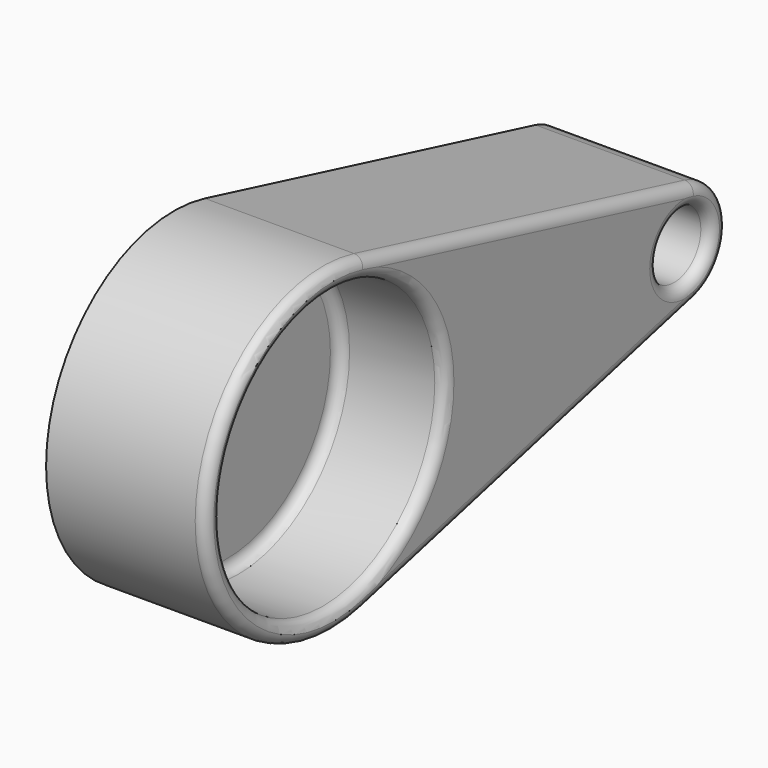
from build123d import *

# Parameters (mm, degrees)
F1_DEPTH    = 76.2
F2_R        = 66.675
F3_DEPTH    = 50.8
F2_R_2      = 15.875
F4_DEPTH    = 50.8
F5_T        = -2.54
F6_T1_DEPTH = 203.2
F6_T3_DEPTH = 203.2
F6_T6_ANGLE = 208.0724869359
F6_T8_ANGLE = 151.9275130641
F7_R        = 5.08
F8_DEPTH    = 25.4


# Not quite as in the source:
# - a fillet or chamfer that OpenCascade refuses, or shapes differently, is made with other operations: its cross-section is extruded or revolved along the edge and cut away or added


with BuildPart() as f1:
    # F0 (on Right) → F1 (new body)
    with BuildSketch(Plane.YZ):
        with BuildLine():
            ThreePointArc((18.4812146278, 73.9248585111), (60.0612543768, 46.8944103565), (76.2, 0))
            ThreePointArc((76.2, 0), (60.0612543768, -46.8944103565), (18.4812146278, -73.9248585111))
            Line((18.4812146278, -73.9248585111), (215.6141706573, -24.6416195037))
            ThreePointArc((215.6141706573, -24.6416195037), (184.0537657814, 0), (215.6141706573, 24.6416195037))
            Line((215.6141706573, 24.6416195037), (18.4812146278, 73.9248585111))
        make_face()
        with BuildLine():
            ThreePointArc((18.4812146278, -73.9248585111), (60.0612543768, -46.8944103565), (76.2, 0))
            ThreePointArc((76.2, 0), (60.0612543768, 46.8944103565), (18.4812146278, 73.9248585111))
            ThreePointArc((18.4812146278, 73.9248585111), (-76.2, 0), (18.4812146278, -73.9248585111))
        make_face()
        with BuildLine():
            ThreePointArc((234.8537657814, 0), (229.474183907, 15.6314701188), (215.6141706573, 24.6416195037))
            ThreePointArc((215.6141706573, 24.6416195037), (184.0537657814, 0), (215.6141706573, -24.6416195037))
            ThreePointArc((215.6141706573, -24.6416195037), (229.474183907, -15.6314701188), (234.8537657814, 0))
        make_face()
    extrude(amount=F1_DEPTH)

    # F2 (on face) → F3 (cut)
    with BuildSketch(Plane.YZ.offset(76.2)):
        Circle(F2_R)
    extrude(amount=-F3_DEPTH, mode=Mode.SUBTRACT)

    # F2 (on face) → F4 (cut)
    with BuildSketch(Plane.YZ.offset(76.2)):
        with Locations((209.4537657814, 0)):
            Circle(F2_R_2)
    extrude(amount=-F4_DEPTH, mode=Mode.SUBTRACT)

    # F5
    f5_openings = [f1.faces().sort_by_distance(p)[0] for p in [
        (0, 57.51924, 0),
    ]]
    offset(amount=F5_T, openings=f5_openings, kind=Kind.INTERSECTION)

    # F6: fillet of radius 5.08 on 6 edges, made by hand

    # F6_s2 → F6_t1 (cut)
    with BuildSketch(Plane(origin=(0, 0, 0), x_dir=(1, 0, 0), z_dir=(0, 0.9701425001, 0.242535625))):
        with BuildLine():
            ThreePointArc((71.12, 76.2), (74.7121024484, 74.7121024484), (76.2, 71.12))
            Line((76.2, 71.12), (76.2, 76.2))
            Line((76.2, 76.2), (71.12, 76.2))
        make_face()
    extrude(amount=F6_T1_DEPTH, mode=Mode.SUBTRACT)

    # F6_s4 → F6_t3 (cut)
    with BuildSketch(Plane(origin=(0, 197.1329560295, -49.2832390074), x_dir=(1, 0, 0), z_dir=(0, -0.9701425001, 0.242535625))):
        with BuildLine():
            ThreePointArc((76.2, 71.12), (74.7121024484, 74.7121024484), (71.12, 76.2))
            Line((71.12, 76.2), (76.2, 76.2))
            Line((76.2, 76.2), (76.2, 71.12))
        make_face()
    extrude(amount=F6_T3_DEPTH, mode=Mode.SUBTRACT)

    # F6_s5 → F6_t6 (revolve, cut)
    with BuildSketch(Plane(origin=(0, 0, 0), x_dir=(1, 0, 0), z_dir=(0, 0.9701425001, -0.242535625))):
        with BuildLine():
            ThreePointArc((71.12, -76.2), (74.7121024484, -74.7121024484), (76.2, -71.12))
            Line((76.2, -71.12), (76.2, -76.2))
            Line((76.2, -76.2), (71.12, -76.2))
        make_face()
    revolve(axis=Axis((76.2, 0, 0), (1, 0, 0)), revolution_arc=F6_T6_ANGLE, mode=Mode.SUBTRACT)

    # F6_s7 → F6_t8 (revolve, cut)
    with BuildSketch(Plane(origin=(0, 197.1329560295, 49.2832390074), x_dir=(1, 0, 0), z_dir=(0, -0.9701425001, -0.242535625))):
        with BuildLine():
            ThreePointArc((71.12, -76.2), (74.7121024484, -74.7121024484), (76.2, -71.12))
            Line((76.2, -71.12), (76.2, -76.2))
            Line((76.2, -76.2), (71.12, -76.2))
        make_face()
    revolve(axis=Axis((76.2, 209.4537657814, 0), (1, 0, 0)), revolution_arc=F6_T8_ANGLE, mode=Mode.SUBTRACT)

    # F6_s9 → F6_t10 (revolve, cut)
    with BuildSketch(Plane.XY):
        with BuildLine():
            ThreePointArc((76.2, 71.755), (74.7121024484, 68.1628975516), (71.12, 66.675))
            Line((71.12, 66.675), (76.2, 66.675))
            Line((76.2, 66.675), (76.2, 71.755))
        make_face()
    revolve(axis=Axis((76.2, 0, 0), (1, 0, 0)), mode=Mode.SUBTRACT)

    # F6_s11 → F6_t12 (revolve, cut)
    with BuildSketch(Plane.XY):
        with BuildLine():
            ThreePointArc((76.2, 230.4087657814), (74.7121024484, 226.8166633329), (71.12, 225.3287657814))
            Line((71.12, 225.3287657814), (76.2, 225.3287657814))
            Line((76.2, 225.3287657814), (76.2, 230.4087657814))
        make_face()
    revolve(axis=Axis((76.2, 209.4537657814, 0), (1, 0, 0)), mode=Mode.SUBTRACT)

    # F7
    f7_edges = [f1.edges().sort_by_distance(p)[0] for p in [
        (25.4, -66.675, 0),
        (25.4, 193.578766, 0),
    ]]
    fillet(f7_edges, radius=F7_R)

    # F8 (add): a face of the model
    f8_faces = [f1.faces().sort_by_distance(p)[0] for p in [
        (22.86, 0, 0),
    ]]
    extrude(f8_faces, amount=F8_DEPTH)


solid = f1.part
